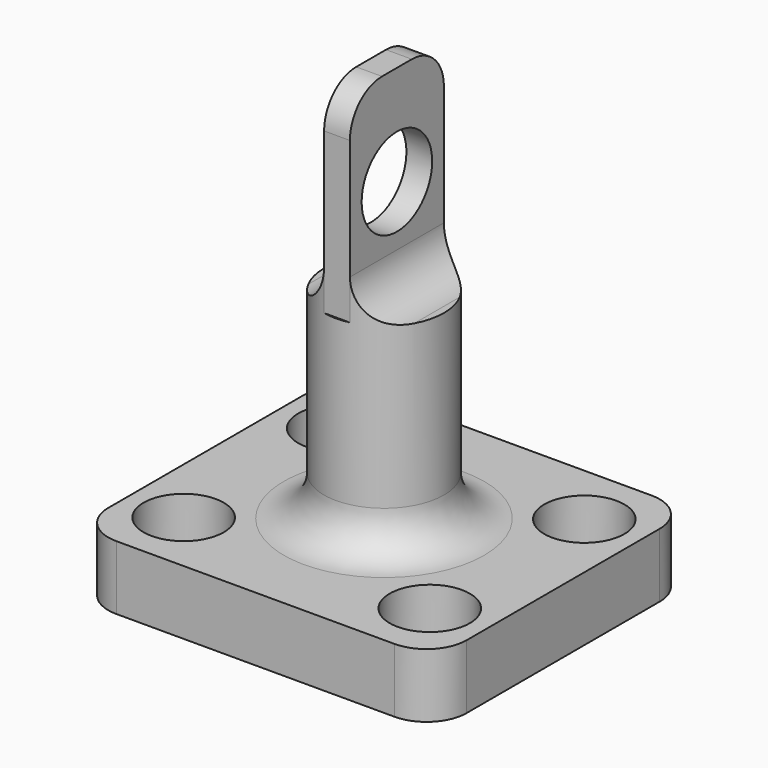
from build123d import *

# Parameters (mm, degrees)
F0_W          = 44.7
F0_H          = 40.1
F0_R          = 5
F1_DEPTH      = 8
F0_R_2        = 4
F2_DEPTH      = 1
F3_R          = 7.5
F4_DEPTH      = 25
F5_W          = 3.2212789527
F5_H          = 14.6500294167
F6_DEPTH      = 25
F7_R          = 5.5
F8_DEPTH      = 10
F9_R          = 5
F10_T4_DEPTH  = 14.6500294167
F10_S5_R      = 7.5
F10_T6_DEPTH  = 10
F10_T10_DEPTH = 14.6500294167
F10_S11_R     = 7.5
F10_T12_DEPTH = 10


# Not quite as in the source:
# - a fillet or chamfer that OpenCascade refuses, or shapes differently, is made with other operations: its cross-section is extruded or revolved along the edge and cut away or added


with BuildPart() as f1:
    # F0 (on Top) → F1 (new body)
    with BuildSketch(Plane.XY):
        Rectangle(F0_W, F0_H)
        with Locations((-15.35, -12.05)):
            Circle(F0_R, mode=Mode.SUBTRACT)
        with Locations((15.35, -12.05)):
            Circle(F0_R, mode=Mode.SUBTRACT)
        with Locations((-15.35, 12.05)):
            Circle(F0_R, mode=Mode.SUBTRACT)
        with Locations((15.35, 12.05)):
            Circle(F0_R, mode=Mode.SUBTRACT)
    extrude(amount=F1_DEPTH)

    # F0 (on Top) → F2 (join)
    with BuildSketch(Plane.XY):
        with Locations((15.35, 12.05)):
            Circle(F0_R)
        with Locations((15.35, 12.05)):
            Circle(F0_R_2, mode=Mode.SUBTRACT)
        with Locations((15.35, -12.05)):
            Circle(F0_R)
        with Locations((15.35, -12.05)):
            Circle(F0_R_2, mode=Mode.SUBTRACT)
        with Locations((-15.35, -12.05)):
            Circle(F0_R)
        with Locations((-15.35, -12.05)):
            Circle(F0_R_2, mode=Mode.SUBTRACT)
        with Locations((-15.35, 12.05)):
            Circle(F0_R)
        with Locations((-15.35, 12.05)):
            Circle(F0_R_2, mode=Mode.SUBTRACT)
    extrude(amount=F2_DEPTH)

    # F3 (on face) → F4 (join)
    with BuildSketch(Plane.XY.offset(8)):
        Circle(F3_R)
    extrude(amount=F4_DEPTH)

    # F5 (on face) → F6 (join)
    with BuildSketch(Plane.XY.offset(33)):
        Rectangle(F5_W, F5_H)
    extrude(amount=F6_DEPTH)

    # F7 (on face) → F8 (cut)
    with BuildSketch(Plane(origin=(-1.6106394764, 0, 0), x_dir=(0, -1, 0), z_dir=(-1, 0, 0))):
        with Locations((0, 45.5)):
            Circle(F7_R)
    extrude(amount=-F8_DEPTH, mode=Mode.SUBTRACT)

    # F9
    f9_edges = [f1.edges().sort_by_distance(p)[0] for p in [
        (0, 7.325015, 58),
        (0, -7.325015, 58),
        (-22.35, 20.05, 4),
        (-22.35, -20.05, 4),
        (22.35, -20.05, 4),
        (22.35, 20.05, 4),
    ]]
    fillet(f9_edges, radius=F9_R)

    # F10: fillet of radius 5 on 3 edges, made by hand


with BuildPart() as f10_tool2:
    # F10_s3 → F10_t4 (new body)
    with BuildSketch(Plane.XZ.offset(7.3250147083)):
        with BuildLine():
            ThreePointArc((6.6106394764, 33), (3.0751055704, 34.4644660941), (1.6106394764, 38))
            Line((1.6106394764, 38), (1.6106394764, 33))
            Line((1.6106394764, 33), (6.6106394764, 33))
        make_face()
    extrude(amount=-F10_T4_DEPTH)

    # F10_s5 → F10_t6 (intersect, symmetric)
    with BuildSketch(Plane.XY.offset(35.5)):
        Circle(F10_S5_R)
    extrude(amount=F10_T6_DEPTH, both=True, mode=Mode.INTERSECT)


with BuildPart() as f1_1:
    add(f1.part)

    # F10_t1: union F10_tool2
    add(f10_tool2.part)


with BuildPart() as f10_tool8:
    # F10_s9 → F10_t10 (new body)
    with BuildSketch(Plane.XZ.offset(-7.3250147083)):
        with BuildLine():
            ThreePointArc((-6.6106394764, 33), (-3.0751055704, 34.4644660941), (-1.6106394764, 38))
            Line((-1.6106394764, 38), (-1.6106394764, 33))
            Line((-1.6106394764, 33), (-6.6106394764, 33))
        make_face()
    extrude(amount=F10_T10_DEPTH)

    # F10_s11 → F10_t12 (intersect, symmetric)
    with BuildSketch(Plane.XY.offset(35.5)):
        Circle(F10_S11_R)
    extrude(amount=F10_T12_DEPTH, both=True, mode=Mode.INTERSECT)


with BuildPart() as f1_2:
    add(f1_1.part)

    # F10_t7: union F10_tool8
    add(f10_tool8.part)

    # F10_s13 → F10_t14 (revolve)
    with BuildSketch(Plane.XZ):
        with BuildLine():
            ThreePointArc((12.5, 8), (8.9644660941, 9.4644660941), (7.5, 13))
            Line((7.5, 13), (7.5, 8))
            Line((7.5, 8), (12.5, 8))
        make_face()
    revolve(axis=Axis((0, 0, 8), (0, 0, 1)))


solid = f1_2.part
